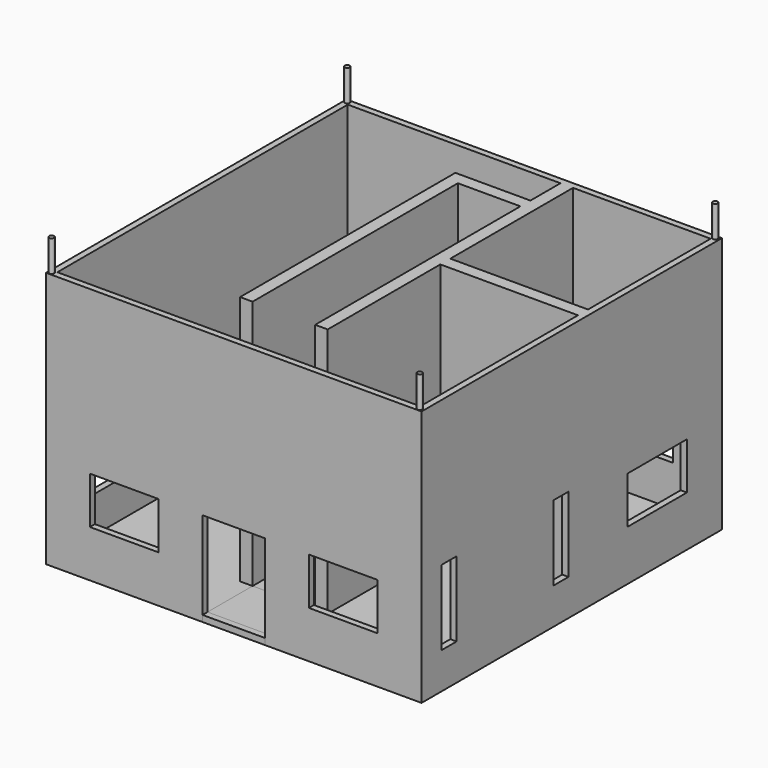
from build123d import *

# Parameters (mm, degrees)
F0_W      = 152.4
F0_H      = 152.4
F1_DEPTH  = 2.54
F2_W      = 152.4
F2_H      = 152.4
F2_W_2    = 147.32
F2_H_2    = 147.32
F3_DEPTH  = 101.6
F4_W      = 25.4
F4_H      = 38.1600596011
F5_DEPTH  = 25.4
F6_W      = 25.4
F6_H      = 22.86
F7_DEPTH  = 2.54
F8_W      = 25.4
F8_H      = 2.54
F9_DEPTH  = 2.54
F11_W     = 5.08
F11_H     = 109.22
F11_H_2   = 124.4600435235
F12_DEPTH = 101.6
F13_W     = 25.4
F13_H     = 5.08
F14_DEPTH = 101.6
F15_W     = 50.8
F15_H     = 35.56
F16_DEPTH = 2.54
F17_W     = 55.8800075936
F17_H     = 5.08
F18_DEPTH = 101.6
F20_DEPTH = 5.08
F22_W     = 7.62
F22_H     = 30.48
F23_DEPTH = 25.4
F24_W     = 30.2523560822
F24_H     = 19.05
F25_DEPTH = 25.4
F21_W     = 27.94
F21_H     = 19.0800298005
F26_DEPTH = 254
F27_DEPTH = 254
F28_W     = 2.5399962032
F28_H     = 5.08
F29_DEPTH = 25.4
F30_W     = 27.94
F30_H     = 19.0754
F31_DEPTH = 25.4
F34_R     = 1.016
F35_DEPTH = 12.7


with BuildPart() as f1:
    # F0 (on Top) → F1 (new body)
    with BuildSketch(Plane.XY):
        with Locations((76.2, -76.2)):
            Rectangle(F0_W, F0_H)
    extrude(amount=F1_DEPTH)

    # F2 (on face) → F3 (join)
    with BuildSketch(Plane.XY.offset(2.54)):
        with Locations((76.2, -76.2)):
            Rectangle(F2_W, F2_H)
        with Locations((76.2, -76.2)):
            Rectangle(F2_W_2, F2_H_2, mode=Mode.SUBTRACT)
    extrude(amount=F3_DEPTH)

    # F4 (on face) → F5 (cut)
    with BuildSketch(Plane.XZ.offset(152.4)):
        with Locations((76.2, 19.0800298005)):
            Rectangle(F4_W, F4_H)
    extrude(amount=-F5_DEPTH, mode=Mode.SUBTRACT)

    # F11 (on face) → F12 (join)
    with BuildSketch(Plane.XY.offset(2.54)):
        with Locations((60.96, -72.39)):
            Rectangle(F11_W, F11_H)
        with Locations((91.4399924064, -64.7699782383)):
            Rectangle(F11_W, F11_H_2)
    extrude(amount=F12_DEPTH)

    # F13 (on face) → F14 (join)
    with BuildSketch(Plane.XY.offset(104.14)):
        with Locations((76.2, -20.32)):
            Rectangle(F13_W, F13_H)
    extrude(amount=-F14_DEPTH)

    # F15 (on face) → F16 (cut)
    with BuildSketch(Plane(origin=(58.42, 0, 0), x_dir=(0, -1, 0), z_dir=(-1, 0, 0))):
        with Locations((72.39, 80.1668018103)):
            Rectangle(F15_W, F15_H)
    extrude(amount=-F16_DEPTH, mode=Mode.SUBTRACT)

    # F17 (on face) → F18 (join)
    with BuildSketch(Plane.XY.offset(104.14)):
        with Locations((121.9199962032, -67.31)):
            Rectangle(F17_W, F17_H)
    extrude(amount=-F18_DEPTH)

    # F19 (on face) → F20 (cut)
    with BuildSketch(Plane.XZ.offset(69.85)):
        Polygon((109.2199962032, 2.54), (121.9199962032, 2.54), (134.6199962032, 2.54), (134.6199962032, 38.1), (109.2199962032, 38.1), align=None)
    extrude(amount=-F20_DEPTH, mode=Mode.SUBTRACT)

    # F22 (on face) → F23 (cut)
    with BuildSketch(Plane.YZ.offset(152.4)):
        with Locations((-138.43, 29.9698188901)):
            Rectangle(F22_W, F22_H)
        with Locations((-81.6729860806, 29.9698188901)):
            Rectangle(F22_W, F22_H)
    extrude(amount=-F23_DEPTH, mode=Mode.SUBTRACT)

    # F24 (on face) → F25 (cut)
    with BuildSketch(Plane.YZ.offset(152.4)):
        with Locations((-32.9061780411, 29.9698188901)):
            Rectangle(F24_W, F24_H)
    extrude(amount=-F25_DEPTH, mode=Mode.SUBTRACT)

    # F21 (on face) → F26 (cut)
    with BuildSketch(Plane.XZ.offset(152.4)):
        with Locations((31.75, 28.6200447008)):
            Rectangle(F21_W, F21_H)
    extrude(amount=-F26_DEPTH, mode=Mode.SUBTRACT)

    # F21 (on face) → F27 (cut)
    with BuildSketch(Plane.XZ.offset(152.4)):
        with Locations((120.65, 28.6200447008)):
            Rectangle(F21_W, F21_H)
    extrude(amount=-F27_DEPTH, mode=Mode.SUBTRACT)

    # F28 (on face) → F29 (join)
    with BuildSketch(Plane.XY.offset(19.0800298005)):
        with Locations((107.9499981016, -67.31)):
            Rectangle(F28_W, F28_H)
    extrude(amount=F29_DEPTH)

    # F30 (on face) → F31 (cut)
    with BuildSketch(Plane(origin=(0, 0, 0), x_dir=(0, -1, 0), z_dir=(-1, 0, 0))):
        with Locations((120.65, 26.8014365758)):
            Rectangle(F30_W, F30_H)
        with Locations((31.75, 26.8014365758)):
            Rectangle(F30_W, F30_H)
    extrude(amount=-F31_DEPTH, mode=Mode.SUBTRACT)

    # F34 (on face) → F35 (join)
    with BuildSketch(Plane.XY.offset(104.14)):
        with Locations((1.2333957711, -151.13)):
            Circle(F34_R)
        with Locations((1.3362482423, -1.27)):
            Circle(F34_R)
        with Locations((150.7363170385, -1.27)):
            Circle(F34_R)
        with Locations((150.6897211075, -151.13)):
            Circle(F34_R)
    extrude(amount=F35_DEPTH)


with BuildPart() as f7:
    # F6 (on face) → F7 (new body)
    with BuildSketch(Plane.XY.offset(2.54)):
        with Locations((76.2, -138.43)):
            Rectangle(F6_W, F6_H)
    extrude(amount=-F7_DEPTH)


with BuildPart() as f9:
    # F8 (on face) → F9 (new body)
    with BuildSketch(Plane.XZ.offset(149.86)):
        with Locations((76.2, 1.27)):
            Rectangle(F8_W, F8_H)
    extrude(amount=F9_DEPTH)


solid = Compound([f1.part, f7.part, f9.part])
